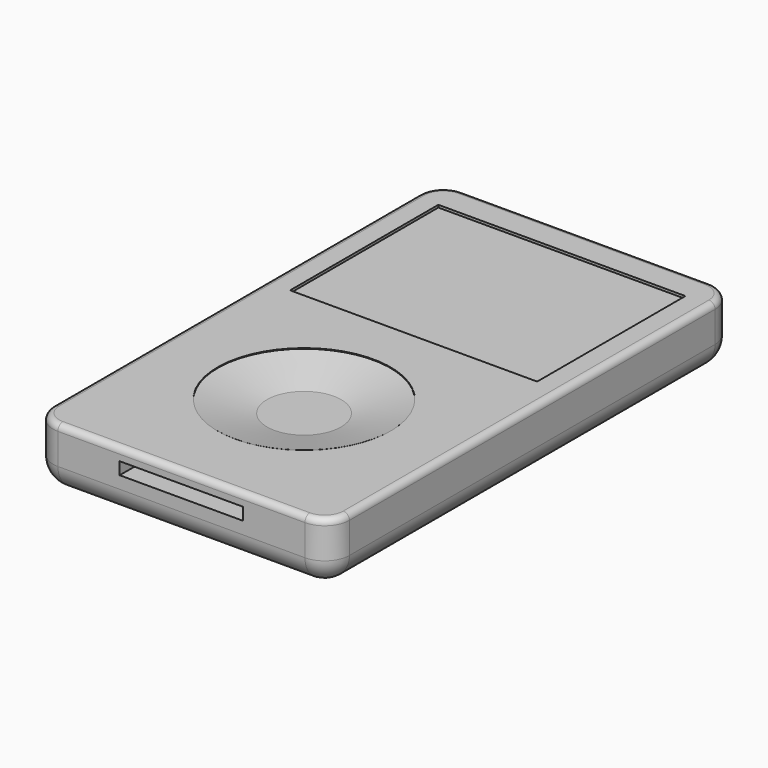
from build123d import *

# Parameters (mm, degrees)
F0_W         = 60.96
F0_H         = 104.14
F0_R         = 17.78
F0_W_2       = 50.8
F0_H_2       = 38.1
F0_R_2       = 7.62
F5_DEPTH     = 12.7
F6_R         = 5.08
F7_R         = 1.27
F8_T1_DEPTH  = 7.62
F8_T4_ANGLE  = 90
F8_S7_W      = 5.08
F8_S7_H      = 5.08
F8_T8_DEPTH  = 5.08
F9_T1_DEPTH  = 7.62
F9_T4_ANGLE  = 90
F9_S7_W      = 5.08
F9_S7_H      = 5.08
F9_T8_DEPTH  = 5.08
F10_T1_DEPTH = 7.62
F10_T4_ANGLE = 90
F10_S7_W     = 5.08
F10_S7_H     = 5.08
F10_T8_DEPTH = 5.08
F11_T1_DEPTH = 7.62
F11_T4_ANGLE = 90
F11_S7_W     = 5.08
F11_S7_H     = 5.08
F11_T8_DEPTH = 5.08
F3_W         = 25.4
F3_H         = 2.54
F12_DEPTH    = 5.08
F4_W         = 9.1439969838
F4_H         = 2.7940007858
F13_DEPTH    = 1.27
F4_R         = 1.8751327249
F14_DEPTH    = 12.7
F17_DEPTH    = 0.508


# Not quite as in the source:
# - a fillet or chamfer that OpenCascade refuses, or shapes differently, is made with other operations: its cross-section is extruded or revolved along the edge and cut away or added


with BuildPart() as f5:
    # F0 (on Top) → F5 (new body)
    with BuildSketch(Plane.XY):
        Rectangle(F0_W, F0_H)
        with Locations((0, -21.59)):
            Circle(F0_R, mode=Mode.SUBTRACT)
        with Locations((0, 26.67)):
            Rectangle(F0_W_2, F0_H_2, mode=Mode.SUBTRACT)
        with Locations((0, 26.67)):
            Rectangle(F0_W_2, F0_H_2)
        with Locations((0, -21.59)):
            Circle(F0_R)
        with Locations((0, -21.59)):
            Circle(F0_R_2, mode=Mode.SUBTRACT)
        with Locations((0, -21.59)):
            Circle(F0_R_2)
    extrude(amount=-F5_DEPTH)

    # F6
    f6_edges = [f5.edges().sort_by_distance(p)[0] for p in [
        (0, -52.07, -12.7),
        (30.48, 0, -12.7),
        (0, 52.07, -12.7),
        (-30.48, 0, -12.7),
    ]]
    fillet(f6_edges, radius=F6_R)

    # F7
    f7_edges = [f5.edges().sort_by_distance(p)[0] for p in [
        (0, -52.07, 0),
        (30.48, 0, 0),
        (0, 52.07, 0),
        (-30.48, 0, 0),
    ]]
    fillet(f7_edges, radius=F7_R)

    # F8: fillet of radius 5.08 on 3 edges, made by hand

    # F8_s2 → F8_t1 (cut)
    with BuildSketch(Plane.XY.offset(-7.62)):
        with BuildLine():
            ThreePointArc((-25.4, -52.07), (-28.9921024484, -50.5821024484), (-30.48, -46.99))
            Line((-30.48, -46.99), (-30.48, -52.07))
            Line((-30.48, -52.07), (-25.4, -52.07))
        make_face()
    extrude(amount=F8_T1_DEPTH, mode=Mode.SUBTRACT)

    # F8_s3 → F8_t4 (revolve, cut)
    with BuildSketch(Plane.XZ.offset(46.99)):
        with BuildLine():
            ThreePointArc((-29.21, 0), (-30.1080256121, -0.3719743879), (-30.48, -1.27))
            Line((-30.48, -1.27), (-30.48, 0))
            Line((-30.48, 0), (-29.21, 0))
        make_face()
    revolve(axis=Axis((-25.4, -46.99, 0), (0, 0, 1)), revolution_arc=F8_T4_ANGLE, mode=Mode.SUBTRACT)


with BuildPart() as f8_tool6:
    # F8_s7 → F8_t8 (new body)
    with BuildSketch(Plane.XZ.offset(46.99)):
        with Locations((-27.94, -10.16)):
            Rectangle(F8_S7_W, F8_S7_H)
    extrude(amount=F8_T8_DEPTH)

    # F8_s9 → F8_t10 (revolve, cut)
    with BuildSketch(Plane(origin=(-25.4, -46.99, -7.62), x_dir=(0.7071067812, 0, 0.7071067812), z_dir=(0.7071067812, 0, -0.7071067812))):
        with BuildLine():
            ThreePointArc((0, -5.08), (5.08, 0), (0, 5.08))
            Line((0, 5.08), (0, -5.08))
        make_face()
    revolve(axis=Axis((-25.4, -46.99, -7.62), (0, -1, 0)), mode=Mode.SUBTRACT)


with BuildPart() as f5_1:
    add(f5.part)

    # F8_t5: cut F8_tool6
    add(f8_tool6.part, mode=Mode.SUBTRACT)

    # F9: fillet of radius 5.08 on 3 edges, made by hand

    # F9_s2 → F9_t1 (cut)
    with BuildSketch(Plane.XY.offset(-7.62)):
        with BuildLine():
            ThreePointArc((25.4, -52.07), (28.9921024484, -50.5821024484), (30.48, -46.99))
            Line((30.48, -46.99), (30.48, -52.07))
            Line((30.48, -52.07), (25.4, -52.07))
        make_face()
    extrude(amount=F9_T1_DEPTH, mode=Mode.SUBTRACT)

    # F9_s3 → F9_t4 (revolve, cut)
    with BuildSketch(Plane.YZ.offset(25.4)):
        with BuildLine():
            ThreePointArc((-50.8, 0), (-51.6980256121, -0.3719743879), (-52.07, -1.27))
            Line((-52.07, -1.27), (-52.07, 0))
            Line((-52.07, 0), (-50.8, 0))
        make_face()
    revolve(axis=Axis((25.4, -46.99, 0), (0, 0, 1)), revolution_arc=F9_T4_ANGLE, mode=Mode.SUBTRACT)


with BuildPart() as f9_tool6:
    # F9_s7 → F9_t8 (new body)
    with BuildSketch(Plane.XZ.offset(46.99)):
        with Locations((27.94, -10.16)):
            Rectangle(F9_S7_W, F9_S7_H)
    extrude(amount=F9_T8_DEPTH)

    # F9_s9 → F9_t10 (revolve, cut)
    with BuildSketch(Plane(origin=(25.4, -46.99, -7.62), x_dir=(-0.7071067812, 0, 0.7071067812), z_dir=(0.7071067812, 0, 0.7071067812))):
        with BuildLine():
            ThreePointArc((0, -5.08), (5.08, 0), (0, 5.08))
            Line((0, 5.08), (0, -5.08))
        make_face()
    revolve(axis=Axis((25.4, -46.99, -7.62), (0, -1, 0)), mode=Mode.SUBTRACT)


with BuildPart() as f5_2:
    add(f5_1.part)

    # F9_t5: cut F9_tool6
    add(f9_tool6.part, mode=Mode.SUBTRACT)

    # F10: fillet of radius 5.08 on 3 edges, made by hand

    # F10_s2 → F10_t1 (cut)
    with BuildSketch(Plane.XY.offset(-7.62)):
        with BuildLine():
            ThreePointArc((30.48, 46.99), (28.9921024484, 50.5821024484), (25.4, 52.07))
            Line((25.4, 52.07), (30.48, 52.07))
            Line((30.48, 52.07), (30.48, 46.99))
        make_face()
    extrude(amount=F10_T1_DEPTH, mode=Mode.SUBTRACT)

    # F10_s3 → F10_t4 (revolve, cut)
    with BuildSketch(Plane.XZ.offset(-46.99)):
        with BuildLine():
            ThreePointArc((29.21, 0), (30.1080256121, -0.3719743879), (30.48, -1.27))
            Line((30.48, -1.27), (30.48, 0))
            Line((30.48, 0), (29.21, 0))
        make_face()
    revolve(axis=Axis((25.4, 46.99, 0), (0, 0, 1)), revolution_arc=F10_T4_ANGLE, mode=Mode.SUBTRACT)


with BuildPart() as f10_tool6:
    # F10_s7 → F10_t8 (new body)
    with BuildSketch(Plane.YZ.offset(25.4)):
        with Locations((49.53, -10.16)):
            Rectangle(F10_S7_W, F10_S7_H)
    extrude(amount=F10_T8_DEPTH)

    # F10_s9 → F10_t10 (revolve, cut)
    with BuildSketch(Plane(origin=(25.4, 46.99, -7.62), x_dir=(0, -0.7071067812, 0.7071067812), z_dir=(0, 0.7071067812, 0.7071067812))):
        with BuildLine():
            ThreePointArc((0, -5.08), (5.08, 0), (0, 5.08))
            Line((0, 5.08), (0, -5.08))
        make_face()
    revolve(axis=Axis((25.4, 46.99, -7.62), (1, 0, 0)), mode=Mode.SUBTRACT)


with BuildPart() as f5_3:
    add(f5_2.part)

    # F10_t5: cut F10_tool6
    add(f10_tool6.part, mode=Mode.SUBTRACT)

    # F11: fillet of radius 5.08 on 3 edges, made by hand

    # F11_s2 → F11_t1 (cut)
    with BuildSketch(Plane.XY.offset(-7.62)):
        with BuildLine():
            ThreePointArc((-30.48, 46.99), (-28.9921024484, 50.5821024484), (-25.4, 52.07))
            Line((-25.4, 52.07), (-30.48, 52.07))
            Line((-30.48, 52.07), (-30.48, 46.99))
        make_face()
    extrude(amount=F11_T1_DEPTH, mode=Mode.SUBTRACT)

    # F11_s3 → F11_t4 (revolve, cut)
    with BuildSketch(Plane.YZ.offset(-25.4)):
        with BuildLine():
            ThreePointArc((50.8, 0), (51.6980256121, -0.3719743879), (52.07, -1.27))
            Line((52.07, -1.27), (52.07, 0))
            Line((52.07, 0), (50.8, 0))
        make_face()
    revolve(axis=Axis((-25.4, 46.99, 0), (0, 0, 1)), revolution_arc=F11_T4_ANGLE, mode=Mode.SUBTRACT)


with BuildPart() as f11_tool6:
    # F11_s7 → F11_t8 (new body)
    with BuildSketch(Plane.YZ.offset(-25.4)):
        with Locations((49.53, -10.16)):
            Rectangle(F11_S7_W, F11_S7_H)
    extrude(amount=-F11_T8_DEPTH)

    # F11_s9 → F11_t10 (revolve, cut)
    with BuildSketch(Plane(origin=(-25.4, 46.99, -7.62), x_dir=(0, -0.7071067812, 0.7071067812), z_dir=(0, -0.7071067812, -0.7071067812))):
        with BuildLine():
            ThreePointArc((0, -5.08), (5.08, 0), (0, 5.08))
            Line((0, 5.08), (0, -5.08))
        make_face()
    revolve(axis=Axis((-25.4, 46.99, -7.62), (-1, 0, 0)), mode=Mode.SUBTRACT)


with BuildPart() as f5_4:
    add(f5_3.part)

    # F11_t5: cut F11_tool6
    add(f11_tool6.part, mode=Mode.SUBTRACT)

    # F3 (on line) → F12 (cut)
    with BuildSketch(Plane.XZ.offset(52.07)):
        with Locations((0, -3.81)):
            Rectangle(F3_W, F3_H)
    extrude(amount=-F12_DEPTH, mode=Mode.SUBTRACT)

    # F4 (on line) → F13 (cut)
    with BuildSketch(Plane.XZ.offset(-52.07)):
        with Locations((-20.4787496477, -3.7782501895)):
            Rectangle(F4_W, F4_H)
    extrude(amount=F13_DEPTH, mode=Mode.SUBTRACT)

    # F4 (on line) → F14 (cut)
    with BuildSketch(Plane.XZ.offset(-52.07)):
        with Locations((17.7482496947, -3.5242501181)):
            Circle(F4_R)
        with Locations((-20.4787496477, -3.7782501895)):
            Rectangle(F4_W, F4_H)
    extrude(amount=F14_DEPTH, mode=Mode.SUBTRACT)

    # F15 (on Right) → F16 (revolve, cut)
    with BuildSketch(Plane.YZ):
        Polygon((-20.5422501868, 5.2387503395), (-38.3222501868, 4.4979169496), (-38.3222501868, -0.1322916101), (-28.1622501868, -2.54), (-20.5422501868, -2.54), align=None)
    revolve(axis=Axis((0, -20.5422501868, 1.3493751698), (0, 0, 1)), mode=Mode.SUBTRACT)

    # F0 (on Top) → F17 (cut)
    with BuildSketch(Plane.XY):
        with Locations((0, 26.67)):
            Rectangle(F0_W_2, F0_H_2)
    extrude(amount=-F17_DEPTH, mode=Mode.SUBTRACT)


solid = f5_4.part
